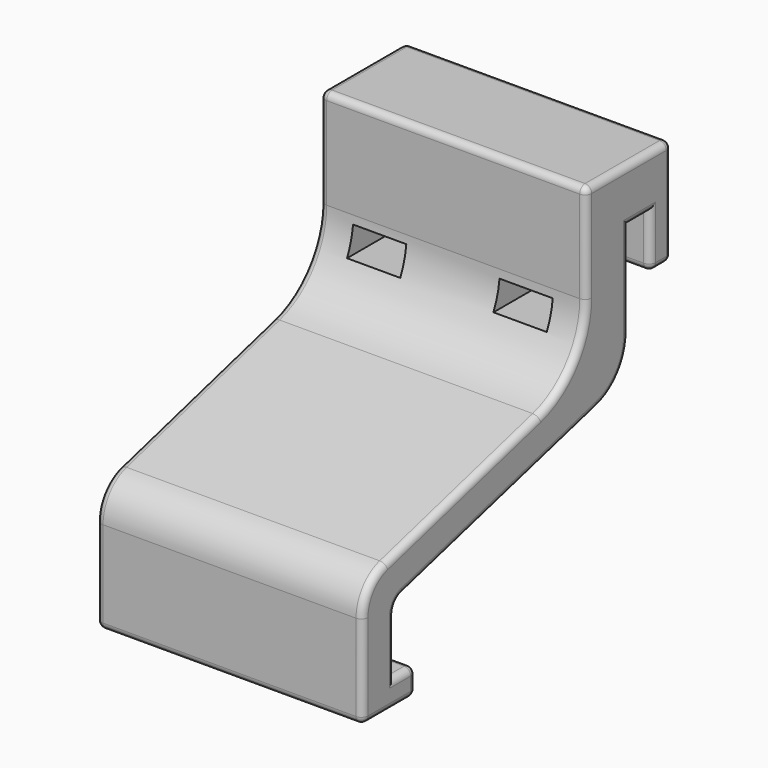
from build123d import *

# Parameters (mm, degrees)
F1_DEPTH = 10
F2_W     = 4
F2_H     = 2
F3_DEPTH = 4.5984521023
F4_R     = 0.5


with BuildPart() as f1:
    # F0 (on Right) → F1 (new body, symmetric)
    with BuildSketch(Plane.YZ):
        with BuildLine():
            Line((0, -7.0358098146), (0, 0))
            Line((0, 0), (2, 0))
            Line((2, 0), (2, -4))
            Line((2, -4), (4, -4))
            Line((4, -4), (4, 0))
            Line((4, 0), (4, 4))
            Line((4, 4), (-4, 4))
            Line((-4, 4), (-4, 0))
            Line((-4, 0), (-4, -3.4128310664))
            ThreePointArc((-4, -3.4128310664), (-5.2334442571, -7.0569971371), (-8.4266487834, -9.2028713037))
            Line((-8.4266487834, -9.2028713037), (-22.7866756083, -13.1049798814))
            ThreePointArc((-22.7866756083, -13.1049798814), (-24.3832778714, -14.1779169647), (-25, -16))
            Line((-25, -16), (-25, -21))
            Line((-25, -21), (-25, -23))
            Line((-25, -23), (-20, -23))
            Line((-20, -23), (-20, -21))
            Line((-20, -21), (-22, -21))
            Line((-22, -21), (-22, -16.767326988))
            ThreePointArc((-22, -16.767326988), (-21.7933533403, -16.158565559), (-21.2588190451, -15.8014011617))
            Line((-21.2588190451, -15.8014011617), (-2.9647238196, -10.8995131198))
            ThreePointArc((-2.9647238196, -10.8995131198), (-0.8265866388, -9.4708555306), (0, -7.0358098146))
        make_face()
    extrude(amount=F1_DEPTH, both=True)

    # F2 (on face) → F3 (cut, through all)
    with BuildSketch(Plane(origin=(0, 0, 0), x_dir=(-1, 0, 0), z_dir=(0, 1, 0))):
        with Locations((-5.5, -5.0229031369)):
            Rectangle(F2_W, F2_H)
        with Locations((5.5, -5.0229031369)):
            Rectangle(F2_W, F2_H)
    extrude(amount=-F3_DEPTH, mode=Mode.SUBTRACT)

    # F4
    f4_edges = [f1.edges().sort_by_distance(p)[0] for p in [
        (10, -5.233444, -7.056997),
        (10, -15.606662, -11.153926),
        (10, -22.5, -23),
        (10, -20, -22),
        (10, -21, -21),
        (10, -22, -18.883663),
        (0, -25, -23),
        (-10, -25, -19.5),
        (0, -4, 4),
        (10, 0, 4),
        (10, 1, 0),
        (10, 2, -2),
        (0, 2, -4),
        (10, 3, -4),
        (10, 4, 0),
        (0, 4, 4),
        (-10, 0, 4),
        (-10, -0.826587, -9.470856),
        (-10, 0, -3.517905),
        (-10, 1, 0),
        (-10, 2, -2),
        (-10, 3, -4),
        (-10, 4, 0),
        (-10, -4, 0.293584),
        (-10, -5.233444, -7.056997),
        (-10, -15.606662, -11.153926),
        (-10, -24.383278, -14.177917),
        (-10, -22.5, -23),
        (-10, -20, -22),
        (-10, -21, -21),
        (-10, -22, -18.883663),
        (-10, -21.793353, -16.158566),
        (-10, -12.111771, -13.350457),
        (10, -24.383278, -14.177917),
        (10, -21.793353, -16.158566),
        (0, -20, -21),
        (0, -20, -23),
        (0, 4, -4),
    ]]
    fillet(f4_edges, radius=F4_R)


solid = f1.part
